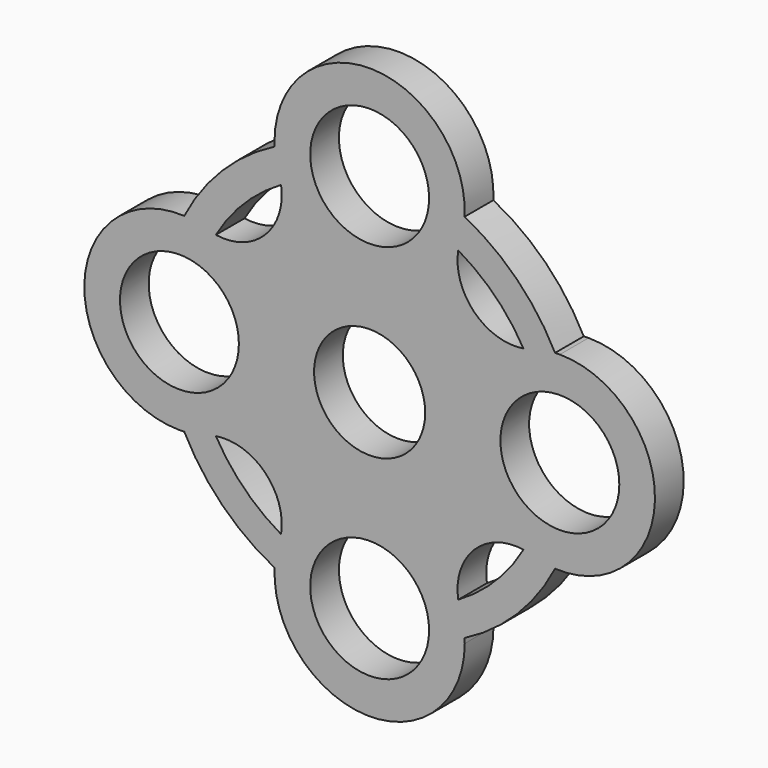
from build123d import *

# Parameters (mm, degrees)
F0_R            = 38.1
F1_DEPTH        = 7.1882
F2_R            = 11.1252
F3_DEPTH        = 7.62
F5_DEPTH        = 7.1882
F5_COPIES_COUNT = 4
F7_DEPTH        = 25.4
F9_DEPTH        = 7.1882
F10_R           = 11.90625
F11_DEPTH       = 25.4


# Not quite as in the source:
# - a pattern or mirror of a feature is missing from the dataset's text; its kind, count and spacing are read off the source's solid


with BuildPart() as f1:
    # F0 (on Front) → F1 (new body)
    with BuildSketch(Plane.XZ):
        Circle(F0_R)
    extrude(amount=F1_DEPTH)

    # F2 (on face) → F3 (cut)
    with BuildSketch(Plane.XZ.offset(7.1882)):
        Circle(F2_R)
    extrude(amount=-F3_DEPTH, mode=Mode.SUBTRACT)

    # F4 (on face) → F5 (join)
    with BuildSketch(Plane.XZ.offset(7.1882)):
        with BuildLine():
            ThreePointArc((-18.4450831863, 33.3375), (0, 19.05), (18.4450831863, 33.3375))
            ThreePointArc((18.4450831863, 33.3375), (0, 38.1), (-18.4450831863, 33.3375))
        make_face()
        with BuildLine():
            ThreePointArc((-19.05, 0), (-23.0396526434, 11.6656949), (-33.3375, 18.4450831863))
            ThreePointArc((-33.3375, 18.4450831863), (-38.1, 0), (-33.3375, -18.4450831863))
            ThreePointArc((-33.3375, -18.4450831863), (-23.0396526434, -11.6656949), (-19.05, 0))
        make_face()
        with BuildLine():
            ThreePointArc((19.05, -38.1), (18.8981657139, -35.6996182282), (18.4450831863, -33.3375))
            ThreePointArc((18.4450831863, -33.3375), (0, -38.1), (-18.4450831863, -33.3375))
            ThreePointArc((-18.4450831863, -33.3375), (-2.4003817718, -56.9981657139), (19.05, -38.1))
        make_face()
        with BuildLine():
            ThreePointArc((38.1, 0), (36.8901663726, 9.525), (33.3375, 18.4450831863))
            ThreePointArc((33.3375, 18.4450831863), (19.05, 0), (33.3375, -18.4450831863))
            ThreePointArc((33.3375, -18.4450831863), (36.8901663726, -9.525), (38.1, 0))
        make_face()
    f5 = extrude(amount=-F5_DEPTH)

    # F5_copies: F5 ×4 about axis
    f5_copies_axis = Axis((0, 0, 0), (0, 1, 0))
    for i in range(1, F5_COPIES_COUNT):
        add(f5.rotate(f5_copies_axis, i * 360 / F5_COPIES_COUNT))

    # F6 (on face) → F7 (cut)
    with BuildSketch(Plane.XZ.offset(7.1882)):
        with BuildLine():
            ThreePointArc((-33.3375, 18.4450831863), (-20.9517399354, 20.9517399354), (-18.4450831863, 33.3375))
            ThreePointArc((-18.4450831863, 33.3375), (-26.9407683632, 26.9407683632), (-33.3375, 18.4450831863))
        make_face()
        with BuildLine():
            ThreePointArc((-18.4450831863, -33.3375), (-20.9517399354, -20.9517399354), (-33.3375, -18.4450831863))
            ThreePointArc((-33.3375, -18.4450831863), (-26.9407683632, -26.9407683632), (-18.4450831863, -33.3375))
        make_face()
        with BuildLine():
            ThreePointArc((18.4450831863, -33.3375), (26.9407683632, -26.9407683632), (33.3375, -18.4450831863))
            ThreePointArc((33.3375, -18.4450831863), (20.9517399354, -20.9517399354), (18.4450831863, -33.3375))
        make_face()
        with BuildLine():
            ThreePointArc((33.3375, 18.4450831863), (26.9407683632, 26.9407683632), (18.4450831863, 33.3375))
            ThreePointArc((18.4450831863, 33.3375), (20.9517399354, 20.9517399354), (33.3375, 18.4450831863))
        make_face()
    extrude(amount=-F7_DEPTH, mode=Mode.SUBTRACT)

    # F8 (on face) → F9 (join)
    with BuildSketch(Plane.XZ.offset(7.1882)):
        with BuildLine():
            ThreePointArc((-37.1387970886, -19.0257349126), (-29.5065148582, -29.5065148582), (-19.0257349126, -37.1387970886))
            ThreePointArc((-19.0257349126, -37.1387970886), (-18.831569694, -35.2234599149), (-18.4450831863, -33.3375))
            ThreePointArc((-18.4450831863, -33.3375), (-18.0201411063, -32.0901876015), (-17.7415806811, -30.8022558951))
            ThreePointArc((-17.7415806811, -30.8022558951), (-25.1350616996, -25.1350616996), (-30.8022558951, -17.7415806811))
            ThreePointArc((-30.8022558951, -17.7415806811), (-32.0901876015, -18.0201411063), (-33.3375, -18.4450831863))
            ThreePointArc((-33.3375, -18.4450831863), (-35.2234599149, -18.831569694), (-37.1387970886, -19.0257349126))
        make_face()
        with BuildLine():
            ThreePointArc((19.0257349126, -37.1387970886), (29.5065148582, -29.5065148582), (37.1387970886, -19.0257349126))
            ThreePointArc((37.1387970886, -19.0257349126), (35.2234599149, -18.831569694), (33.3375, -18.4450831863))
            ThreePointArc((33.3375, -18.4450831863), (32.0901876015, -18.0201411063), (30.8022558951, -17.7415806811))
            ThreePointArc((30.8022558951, -17.7415806811), (25.1350616996, -25.1350616996), (17.7415806811, -30.8022558951))
            ThreePointArc((17.7415806811, -30.8022558951), (18.0201411063, -32.0901876015), (18.4450831863, -33.3375))
            ThreePointArc((18.4450831863, -33.3375), (18.831569694, -35.2234599149), (19.0257349126, -37.1387970886))
        make_face()
        with BuildLine():
            ThreePointArc((33.3375, 18.4450831863), (35.2234599149, 18.831569694), (37.1387970886, 19.0257349126))
            ThreePointArc((37.1387970886, 19.0257349126), (29.5065148582, 29.5065148582), (19.0257349126, 37.1387970886))
            ThreePointArc((19.0257349126, 37.1387970886), (18.831569694, 35.2234599149), (18.4450831863, 33.3375))
            ThreePointArc((18.4450831863, 33.3375), (18.0201411063, 32.0901876015), (17.7415806811, 30.8022558951))
            ThreePointArc((17.7415806811, 30.8022558951), (25.1350616996, 25.1350616996), (30.8022558951, 17.7415806811))
            ThreePointArc((30.8022558951, 17.7415806811), (32.0901876015, 18.0201411063), (33.3375, 18.4450831863))
        make_face()
        with BuildLine():
            ThreePointArc((-18.4450831863, 33.3375), (-18.831569694, 35.2234599149), (-19.0257349126, 37.1387970886))
            ThreePointArc((-19.0257349126, 37.1387970886), (-29.5065148582, 29.5065148582), (-37.1387970886, 19.0257349126))
            ThreePointArc((-37.1387970886, 19.0257349126), (-35.2234599149, 18.831569694), (-33.3375, 18.4450831863))
            ThreePointArc((-33.3375, 18.4450831863), (-32.0901876015, 18.0201411063), (-30.8022558951, 17.7415806811))
            ThreePointArc((-30.8022558951, 17.7415806811), (-25.1350616996, 25.1350616996), (-17.7415806811, 30.8022558951))
            ThreePointArc((-17.7415806811, 30.8022558951), (-18.0201411063, 32.0901876015), (-18.4450831863, 33.3375))
        make_face()
    extrude(amount=-F9_DEPTH)

    # F10 (on face) → F11 (cut)
    with BuildSketch(Plane.XZ.offset(7.1882)):
        with Locations((-38.1, 0)):
            Circle(F10_R)
        with Locations((0, 38.1)):
            Circle(F10_R)
        with Locations((38.1, 0)):
            Circle(F10_R)
        with Locations((0, -38.1)):
            Circle(F10_R)
    extrude(amount=-F11_DEPTH, mode=Mode.SUBTRACT)


solid = f1.part
